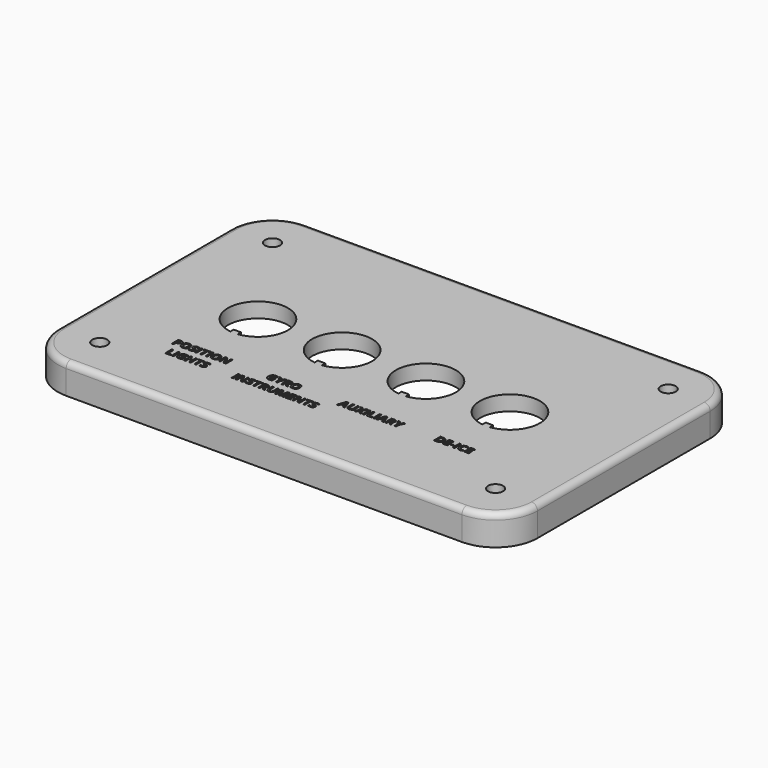
from build123d import *

# Parameters (mm, degrees)
F0_R         = 1.5875
F0_W         = 0.3738893229
F0_H         = 1.7629518229
F0_W_2       = 0.6474574653
F0_H_2       = 0.3013493924
F0_W_3       = 83.82
F0_H_3       = 3.175
F0_TEXT_SIZE = 2.4694444444
F1_DEPTH     = 6.35
F2_R         = 1.27
F3_DEPTH     = 0.508
F5_DEPTH     = 3.175
F6_W         = 83.82
F6_H         = 3.048
F7_DEPTH     = 3.175


# Not quite as in the source:
# - Text() gives the source's letters only with a copy of the font that has no kerning and outlines rounded to 1/6400 em; it was checked with that copy


with BuildPart() as f1:
    # F0 (on Top) → F1 (new body)
    with BuildSketch(Plane.XY):
        with BuildLine():
            Line((-47.7400784737, 22.8871895512), (-47.7400784737, -22.8328104488))
            ThreePointArc((-47.7400784737, -22.8328104488), (-46.0661937282, -26.8739257033), (-42.0250784737, -28.5478104488))
            Line((-42.0250784737, -28.5478104488), (41.7949215263, -28.5478104488))
            ThreePointArc((41.7949215263, -28.5478104488), (45.8360367808, -26.8739257033), (47.5099215263, -22.8328104488))
            Line((47.5099215263, -22.8328104488), (47.5099215263, 22.8871895512))
            ThreePointArc((47.5099215263, 22.8871895512), (45.8360367808, 26.9283048057), (41.7949215263, 28.6021895512))
            Line((41.7949215263, 28.6021895512), (-42.0250784737, 28.6021895512))
            ThreePointArc((-42.0250784737, 28.6021895512), (-46.0661937282, 26.9283048057), (-47.7400784737, 22.8871895512))
        make_face()
        with Locations((-42.0250784737, -22.8328104488)):
            Circle(F0_R, mode=Mode.SUBTRACT)
        Polygon((-30.0736846576, -19.1064444444), (-31.1625553173, -19.1064444444), (-31.1625553173, -17.3434926215), (-30.7886659944, -17.3434926215), (-30.7886659944, -18.7977638889), (-30.0736846576, -18.7977638889), align=None, mode=Mode.SUBTRACT)
        with Locations((-29.5803745447, -18.224968533)):
            Rectangle(F0_W, F0_H, mode=Mode.SUBTRACT)
        with BuildLine():
            Line((-28.2806364805, -18.4277330729), (-28.2806364805, -18.1163515625))
            Line((-28.2806364805, -18.1163515625), (-27.5810891715, -18.1163515625))
            Line((-27.5810891715, -18.1163515625), (-27.5810891715, -19.0304318576))
            add(Edge.make_bspline(
                [(-27.5810891715, -19.0304318576), (-27.7512493277, -19.0859943576), (-27.9013452479, -19.1083736979)],
                knots=[0, 0, 0, 1, 1, 1], degree=2))
            add(Edge.make_bspline(
                [(-27.9013452479, -19.1083736979), (-28.051441168, -19.1307530382), (-28.2080965499, -19.1307530382)],
                knots=[0, 0, 0, 1, 1, 1], degree=2))
            add(Edge.make_bspline(
                [(-28.2080965499, -19.1307530382), (-28.607066168, -19.1307530382), (-28.8175477218, -18.896155816)],
                knots=[0, 0, 0, 1, 1, 1], degree=2))
            add(Edge.make_bspline(
                [(-28.8175477218, -18.896155816), (-29.0280292756, -18.6615585938), (-29.0280292756, -18.2224605035)],
                knots=[0, 0, 0, 1, 1, 1], degree=2))
            add(Edge.make_bspline(
                [(-29.0280292756, -18.2224605035), (-29.0280292756, -17.7957096354), (-28.7837857861, -17.5570609809)],
                knots=[0, 0, 0, 1, 1, 1], degree=2))
            add(Edge.make_bspline(
                [(-28.7837857861, -17.5570609809), (-28.5395422965, -17.3184123264), (-28.107003668, -17.3184123264)],
                knots=[0, 0, 0, 1, 1, 1], degree=2))
            add(Edge.make_bspline(
                [(-28.107003668, -17.3184123264), (-27.8353647791, -17.3184123264), (-27.5834042756, -17.4268363715)],
                knots=[0, 0, 0, 1, 1, 1], degree=2))
            Line((-27.5834042756, -17.4268363715), (-27.7076481993, -17.7258706597))
            add(Edge.make_bspline(
                [(-27.7076481993, -17.7258706597), (-27.9005735465, -17.6294079861), (-28.1093187722, -17.6294079861)],
                knots=[0, 0, 0, 1, 1, 1], degree=2))
            add(Edge.make_bspline(
                [(-28.1093187722, -17.6294079861), (-28.3516330083, -17.6294079861), (-28.4974845708, -17.7922369792)],
                knots=[0, 0, 0, 1, 1, 1], degree=2))
            add(Edge.make_bspline(
                [(-28.4974845708, -17.7922369792), (-28.6433361333, -17.9550659722), (-28.6433361333, -18.2297916667)],
                knots=[0, 0, 0, 1, 1, 1], degree=2))
            add(Edge.make_bspline(
                [(-28.6433361333, -18.2297916667), (-28.6433361333, -18.5168645833), (-28.5258445968, -18.6681180556)],
                knots=[0, 0, 0, 1, 1, 1], degree=2))
            add(Edge.make_bspline(
                [(-28.5258445968, -18.6681180556), (-28.4083530604, -18.8193715278), (-28.1841738069, -18.8193715278)],
                knots=[0, 0, 0, 1, 1, 1], degree=2))
            add(Edge.make_bspline(
                [(-28.1841738069, -18.8193715278), (-28.0668751958, -18.8193715278), (-27.9464897791, -18.7954487847)],
                knots=[0, 0, 0, 1, 1, 1], degree=2))
            Line((-27.9464897791, -18.7954487847), (-27.9464897791, -18.4277330729))
            Line((-27.9464897791, -18.4277330729), (-28.2806364805, -18.4277330729))
        make_face(mode=Mode.SUBTRACT)
        Polygon((-25.7170444666, -17.3434926215), (-25.7170444666, -19.1064444444), (-26.0897762374, -19.1064444444), (-26.0897762374, -18.345546875), (-26.7877801437, -18.345546875), (-26.7877801437, -19.1064444444), (-27.1616694666, -19.1064444444), (-27.1616694666, -17.3434926215), (-26.7877801437, -17.3434926215), (-26.7877801437, -18.0345512153), (-26.0897762374, -18.0345512153), (-26.0897762374, -17.3434926215), align=None, mode=Mode.SUBTRACT)
        Polygon((-24.5919038416, -17.6544882813), (-24.5919038416, -19.1064444444), (-24.9657931645, -19.1064444444), (-24.9657931645, -17.6544882813), (-25.4446338763, -17.6544882813), (-25.4446338763, -17.3434926215), (-24.1134489805, -17.3434926215), (-24.1134489805, -17.6544882813), align=None, mode=Mode.SUBTRACT)
        with BuildLine():
            add(Edge.make_bspline(
                [(-22.8931961593, -18.3256755642), (-22.8015566194, -18.4443246528), (-22.8015566194, -18.6167999132)],
                knots=[0, 0, 0, 1, 1, 1], degree=2))
            add(Edge.make_bspline(
                [(-22.8015566194, -18.6167999132), (-22.8015566194, -18.8556414931), (-22.9734531038, -18.9931972656)],
                knots=[0, 0, 0, 1, 1, 1], degree=2))
            add(Edge.make_bspline(
                [(-22.9734531038, -18.9931972656), (-23.1453495881, -19.1307530382), (-23.4513291888, -19.1307530382)],
                knots=[0, 0, 0, 1, 1, 1], degree=2))
            add(Edge.make_bspline(
                [(-23.4513291888, -19.1307530382), (-23.7337718972, -19.1307530382), (-23.9506199874, -19.0242582465)],
                knots=[0, 0, 0, 1, 1, 1], degree=2))
            Line((-23.9506199874, -19.0242582465), (-23.9506199874, -18.6769926215))
            add(Edge.make_bspline(
                [(-23.9506199874, -18.6769926215), (-23.7723569666, -18.7568637153), (-23.648691819, -18.7892751736)],
                knots=[0, 0, 0, 1, 1, 1], degree=2))
            add(Edge.make_bspline(
                [(-23.648691819, -18.7892751736), (-23.5250266715, -18.8216866319), (-23.4223903868, -18.8216866319)],
                knots=[0, 0, 0, 1, 1, 1], degree=2))
            add(Edge.make_bspline(
                [(-23.4223903868, -18.8216866319), (-23.2996898659, -18.8216866319), (-23.2339023225, -18.7748057726)],
                knots=[0, 0, 0, 1, 1, 1], degree=2))
            add(Edge.make_bspline(
                [(-23.2339023225, -18.7748057726), (-23.1681147791, -18.7279249132), (-23.1681147791, -18.6349348958)],
                knots=[0, 0, 0, 1, 1, 1], degree=2))
            add(Edge.make_bspline(
                [(-23.1681147791, -18.6349348958), (-23.1681147791, -18.5832309028), (-23.1970535812, -18.5427165799)],
                knots=[0, 0, 0, 1, 1, 1], degree=2))
            add(Edge.make_bspline(
                [(-23.1970535812, -18.5427165799), (-23.2259923833, -18.5022022569), (-23.2821336593, -18.4649676649)],
                knots=[0, 0, 0, 1, 1, 1], degree=2))
            add(Edge.make_bspline(
                [(-23.2821336593, -18.4649676649), (-23.3382749354, -18.4277330729), (-23.5107501958, -18.345546875)],
                knots=[0, 0, 0, 1, 1, 1], degree=2))
            add(Edge.make_bspline(
                [(-23.5107501958, -18.345546875), (-23.6720357861, -18.2695342882), (-23.7528715065, -18.1996953125)],
                knots=[0, 0, 0, 1, 1, 1], degree=2))
            add(Edge.make_bspline(
                [(-23.7528715065, -18.1996953125), (-23.833707227, -18.1298563368), (-23.8819385638, -18.0368663194)],
                knots=[0, 0, 0, 1, 1, 1], degree=2))
            add(Edge.make_bspline(
                [(-23.8819385638, -18.0368663194), (-23.9301699006, -17.9438763021), (-23.9301699006, -17.8200182292)],
                knots=[0, 0, 0, 1, 1, 1], degree=2))
            add(Edge.make_bspline(
                [(-23.9301699006, -17.8200182292), (-23.9301699006, -17.5858068576), (-23.7715852652, -17.452109592)],
                knots=[0, 0, 0, 1, 1, 1], degree=2))
            add(Edge.make_bspline(
                [(-23.7715852652, -17.452109592), (-23.6130006298, -17.3184123264), (-23.3332588763, -17.3184123264)],
                knots=[0, 0, 0, 1, 1, 1], degree=2))
            add(Edge.make_bspline(
                [(-23.3332588763, -17.3184123264), (-23.1958960291, -17.3184123264), (-23.0710733295, -17.3508237847)],
                knots=[0, 0, 0, 1, 1, 1], degree=2))
            add(Edge.make_bspline(
                [(-23.0710733295, -17.3508237847), (-22.9462506298, -17.3832352431), (-22.8100453347, -17.4422703993)],
                knots=[0, 0, 0, 1, 1, 1], degree=2))
            Line((-22.8100453347, -17.4422703993), (-22.9304307513, -17.7332018229))
            add(Edge.make_bspline(
                [(-22.9304307513, -17.7332018229), (-23.0716521055, -17.6753242188), (-23.1638704215, -17.6523661024)],
                knots=[0, 0, 0, 1, 1, 1], degree=2))
            add(Edge.make_bspline(
                [(-23.1638704215, -17.6523661024), (-23.2560887374, -17.6294079861), (-23.3452202479, -17.6294079861)],
                knots=[0, 0, 0, 1, 1, 1], degree=2))
            add(Edge.make_bspline(
                [(-23.3452202479, -17.6294079861), (-23.4513291888, -17.6294079861), (-23.5080492409, -17.678796875)],
                knots=[0, 0, 0, 1, 1, 1], degree=2))
            add(Edge.make_bspline(
                [(-23.5080492409, -17.678796875), (-23.564769293, -17.7281857639), (-23.564769293, -17.8076710069)],
                knots=[0, 0, 0, 1, 1, 1], degree=2))
            add(Edge.make_bspline(
                [(-23.564769293, -17.8076710069), (-23.564769293, -17.8570598958), (-23.5418111767, -17.8939086372)],
                knots=[0, 0, 0, 1, 1, 1], degree=2))
            add(Edge.make_bspline(
                [(-23.5418111767, -17.8939086372), (-23.5188530604, -17.9307573785), (-23.4688853954, -17.9650980903)],
                knots=[0, 0, 0, 1, 1, 1], degree=2))
            add(Edge.make_bspline(
                [(-23.4688853954, -17.9650980903), (-23.4189177305, -17.9994388021), (-23.2321659944, -18.0885703125)],
                knots=[0, 0, 0, 1, 1, 1], degree=2))
            add(Edge.make_bspline(
                [(-23.2321659944, -18.0885703125), (-22.9848356993, -18.2070264757), (-22.8931961593, -18.3256755642)],
                knots=[0, 0, 0, 1, 1, 1], degree=2))
        make_face(mode=Mode.SUBTRACT)
        with Locations((-16.8888935736, -18.224968533)):
            Rectangle(F0_W, F0_H, mode=Mode.SUBTRACT)
        with BuildLine():
            Line((-14.694367749, -17.3434926215), (-14.694367749, -19.1064444444))
            Line((-14.694367749, -19.1064444444), (-15.1693499538, -19.1064444444))
            Line((-15.1693499538, -19.1064444444), (-15.9364211344, -17.7729444444))
            Line((-15.9364211344, -17.7729444444), (-15.9472249538, -17.7729444444))
            add(Edge.make_bspline(
                [(-15.9472249538, -17.7729444444), (-15.9240739122, -18.1259978299), (-15.9240739122, -18.2768654514)],
                knots=[0, 0, 0, 1, 1, 1], degree=2))
            Line((-15.9240739122, -18.2768654514), (-15.9240739122, -19.1064444444))
            Line((-15.9240739122, -19.1064444444), (-16.2582206136, -19.1064444444))
            Line((-16.2582206136, -19.1064444444), (-16.2582206136, -17.3434926215))
            Line((-16.2582206136, -17.3434926215), (-15.7867110649, -17.3434926215))
            Line((-15.7867110649, -17.3434926215), (-15.0211832872, -18.6638736979))
            Line((-15.0211832872, -18.6638736979), (-15.0126945719, -18.6638736979))
            add(Edge.make_bspline(
                [(-15.0126945719, -18.6638736979), (-15.0308295545, -18.3200807292), (-15.0308295545, -18.1780876736)],
                knots=[0, 0, 0, 1, 1, 1], degree=2))
            Line((-15.0308295545, -18.1780876736), (-15.0308295545, -17.3434926215))
            Line((-15.0308295545, -17.3434926215), (-14.694367749, -17.3434926215))
        make_face(mode=Mode.SUBTRACT)
        with BuildLine():
            add(Edge.make_bspline(
                [(-13.3016396674, -18.3256755642), (-13.2100001274, -18.4443246528), (-13.2100001274, -18.6167999132)],
                knots=[0, 0, 0, 1, 1, 1], degree=2))
            add(Edge.make_bspline(
                [(-13.2100001274, -18.6167999132), (-13.2100001274, -18.8556414931), (-13.3818966118, -18.9931972656)],
                knots=[0, 0, 0, 1, 1, 1], degree=2))
            add(Edge.make_bspline(
                [(-13.3818966118, -18.9931972656), (-13.5537930962, -19.1307530382), (-13.8597726969, -19.1307530382)],
                knots=[0, 0, 0, 1, 1, 1], degree=2))
            add(Edge.make_bspline(
                [(-13.8597726969, -19.1307530382), (-14.1422154052, -19.1307530382), (-14.3590634955, -19.0242582465)],
                knots=[0, 0, 0, 1, 1, 1], degree=2))
            Line((-14.3590634955, -19.0242582465), (-14.3590634955, -18.6769926215))
            add(Edge.make_bspline(
                [(-14.3590634955, -18.6769926215), (-14.1808004747, -18.7568637153), (-14.0571353271, -18.7892751736)],
                knots=[0, 0, 0, 1, 1, 1], degree=2))
            add(Edge.make_bspline(
                [(-14.0571353271, -18.7892751736), (-13.9334701795, -18.8216866319), (-13.8308338948, -18.8216866319)],
                knots=[0, 0, 0, 1, 1, 1], degree=2))
            add(Edge.make_bspline(
                [(-13.8308338948, -18.8216866319), (-13.708133374, -18.8216866319), (-13.6423458306, -18.7748057726)],
                knots=[0, 0, 0, 1, 1, 1], degree=2))
            add(Edge.make_bspline(
                [(-13.6423458306, -18.7748057726), (-13.5765582872, -18.7279249132), (-13.5765582872, -18.6349348958)],
                knots=[0, 0, 0, 1, 1, 1], degree=2))
            add(Edge.make_bspline(
                [(-13.5765582872, -18.6349348958), (-13.5765582872, -18.5832309028), (-13.6054970893, -18.5427165799)],
                knots=[0, 0, 0, 1, 1, 1], degree=2))
            add(Edge.make_bspline(
                [(-13.6054970893, -18.5427165799), (-13.6344358913, -18.5022022569), (-13.6905771674, -18.4649676649)],
                knots=[0, 0, 0, 1, 1, 1], degree=2))
            add(Edge.make_bspline(
                [(-13.6905771674, -18.4649676649), (-13.7467184434, -18.4277330729), (-13.9191937038, -18.345546875)],
                knots=[0, 0, 0, 1, 1, 1], degree=2))
            add(Edge.make_bspline(
                [(-13.9191937038, -18.345546875), (-14.0804792941, -18.2695342882), (-14.1613150146, -18.1996953125)],
                knots=[0, 0, 0, 1, 1, 1], degree=2))
            add(Edge.make_bspline(
                [(-14.1613150146, -18.1996953125), (-14.2421507351, -18.1298563368), (-14.2903820719, -18.0368663194)],
                knots=[0, 0, 0, 1, 1, 1], degree=2))
            add(Edge.make_bspline(
                [(-14.2903820719, -18.0368663194), (-14.3386134087, -17.9438763021), (-14.3386134087, -17.8200182292)],
                knots=[0, 0, 0, 1, 1, 1], degree=2))
            add(Edge.make_bspline(
                [(-14.3386134087, -17.8200182292), (-14.3386134087, -17.5858068576), (-14.1800287733, -17.452109592)],
                knots=[0, 0, 0, 1, 1, 1], degree=2))
            add(Edge.make_bspline(
                [(-14.1800287733, -17.452109592), (-14.0214441379, -17.3184123264), (-13.7417023844, -17.3184123264)],
                knots=[0, 0, 0, 1, 1, 1], degree=2))
            add(Edge.make_bspline(
                [(-13.7417023844, -17.3184123264), (-13.6043395372, -17.3184123264), (-13.4795168375, -17.3508237847)],
                knots=[0, 0, 0, 1, 1, 1], degree=2))
            add(Edge.make_bspline(
                [(-13.4795168375, -17.3508237847), (-13.3546941379, -17.3832352431), (-13.2184888427, -17.4422703993)],
                knots=[0, 0, 0, 1, 1, 1], degree=2))
            Line((-13.2184888427, -17.4422703993), (-13.3388742594, -17.7332018229))
            add(Edge.make_bspline(
                [(-13.3388742594, -17.7332018229), (-13.4800956136, -17.6753242188), (-13.5723139295, -17.6523661024)],
                knots=[0, 0, 0, 1, 1, 1], degree=2))
            add(Edge.make_bspline(
                [(-13.5723139295, -17.6523661024), (-13.6645322455, -17.6294079861), (-13.7536637559, -17.6294079861)],
                knots=[0, 0, 0, 1, 1, 1], degree=2))
            add(Edge.make_bspline(
                [(-13.7536637559, -17.6294079861), (-13.8597726969, -17.6294079861), (-13.916492749, -17.678796875)],
                knots=[0, 0, 0, 1, 1, 1], degree=2))
            add(Edge.make_bspline(
                [(-13.916492749, -17.678796875), (-13.9732128011, -17.7281857639), (-13.9732128011, -17.8076710069)],
                knots=[0, 0, 0, 1, 1, 1], degree=2))
            add(Edge.make_bspline(
                [(-13.9732128011, -17.8076710069), (-13.9732128011, -17.8570598958), (-13.9502546847, -17.8939086372)],
                knots=[0, 0, 0, 1, 1, 1], degree=2))
            add(Edge.make_bspline(
                [(-13.9502546847, -17.8939086372), (-13.9272965684, -17.9307573785), (-13.8773289035, -17.9650980903)],
                knots=[0, 0, 0, 1, 1, 1], degree=2))
            add(Edge.make_bspline(
                [(-13.8773289035, -17.9650980903), (-13.8273612386, -17.9994388021), (-13.6406095024, -18.0885703125)],
                knots=[0, 0, 0, 1, 1, 1], degree=2))
            add(Edge.make_bspline(
                [(-13.6406095024, -18.0885703125), (-13.3932792073, -18.2070264757), (-13.3016396674, -18.3256755642)],
                knots=[0, 0, 0, 1, 1, 1], degree=2))
        make_face(mode=Mode.SUBTRACT)
        Polygon((-12.2102609781, -17.6544882813), (-12.2102609781, -19.1064444444), (-12.5841503011, -19.1064444444), (-12.5841503011, -17.6544882813), (-13.0629910129, -17.6544882813), (-13.0629910129, -17.3434926215), (-11.731806117, -17.3434926215), (-11.731806117, -17.6544882813), align=None, mode=Mode.SUBTRACT)
        with BuildLine():
            Line((-10.8879506483, -18.4300481771), (-11.0866637559, -18.4300481771))
            Line((-11.0866637559, -18.4300481771), (-11.0866637559, -19.1064444444))
            Line((-11.0866637559, -19.1064444444), (-11.4605530788, -19.1064444444))
            Line((-11.4605530788, -19.1064444444), (-11.4605530788, -17.3434926215))
            Line((-11.4605530788, -17.3434926215), (-10.9469858045, -17.3434926215))
            add(Edge.make_bspline(
                [(-10.9469858045, -17.3434926215), (-10.5873729573, -17.3434926215), (-10.4150906222, -17.4742960069)],
                knots=[0, 0, 0, 1, 1, 1], degree=2))
            add(Edge.make_bspline(
                [(-10.4150906222, -17.4742960069), (-10.2428082872, -17.6050993924), (-10.2428082872, -17.8717222222)],
                knots=[0, 0, 0, 1, 1, 1], degree=2))
            add(Edge.make_bspline(
                [(-10.2428082872, -17.8717222222), (-10.2428082872, -18.0272200521), (-10.328274216, -18.1483771701)],
                knots=[0, 0, 0, 1, 1, 1], degree=2))
            add(Edge.make_bspline(
                [(-10.328274216, -18.1483771701), (-10.4137401448, -18.2695342882), (-10.5707813774, -18.3382157118)],
                knots=[0, 0, 0, 1, 1, 1], degree=2))
            add(Edge.make_bspline(
                [(-10.5707813774, -18.3382157118), (-10.1725834608, -18.9328116319), (-10.0521980441, -19.1064444444)],
                knots=[0, 0, 0, 1, 1, 1], degree=2))
            Line((-10.0521980441, -19.1064444444), (-10.4669875406, -19.1064444444))
            Line((-10.4669875406, -19.1064444444), (-10.8879506483, -18.4300481771))
        make_face(mode=Mode.SUBTRACT)
        with BuildLine():
            Line((-8.768086933, -17.3434926215), (-8.3953551622, -17.3434926215))
            Line((-8.3953551622, -17.3434926215), (-8.3953551622, -18.4840672743))
            add(Edge.make_bspline(
                [(-8.3953551622, -18.4840672743), (-8.3953551622, -18.6796935764), (-8.4827503445, -18.826702691)],
                knots=[0, 0, 0, 1, 1, 1], degree=2))
            add(Edge.make_bspline(
                [(-8.4827503445, -18.826702691), (-8.5701455268, -18.9737118056), (-8.7354825493, -19.0522324219)],
                knots=[0, 0, 0, 1, 1, 1], degree=2))
            add(Edge.make_bspline(
                [(-8.7354825493, -19.0522324219), (-8.9008195719, -19.1307530382), (-9.1261563774, -19.1307530382)],
                knots=[0, 0, 0, 1, 1, 1], degree=2))
            add(Edge.make_bspline(
                [(-9.1261563774, -19.1307530382), (-9.4660908393, -19.1307530382), (-9.6541930528, -18.9563485243)],
                knots=[0, 0, 0, 1, 1, 1], degree=2))
            add(Edge.make_bspline(
                [(-9.6541930528, -18.9563485243), (-9.8422952663, -18.7819440104), (-9.8422952663, -18.479437066)],
                knots=[0, 0, 0, 1, 1, 1], degree=2))
            Line((-9.8422952663, -18.479437066), (-9.8422952663, -17.3434926215))
            Line((-9.8422952663, -17.3434926215), (-9.4699493462, -17.3434926215))
            Line((-9.4699493462, -17.3434926215), (-9.4699493462, -18.4227170139))
            add(Edge.make_bspline(
                [(-9.4699493462, -18.4227170139), (-9.4699493462, -18.6264461806), (-9.3879560736, -18.7217513021)],
                knots=[0, 0, 0, 1, 1, 1], degree=2))
            add(Edge.make_bspline(
                [(-9.3879560736, -18.7217513021), (-9.3059628011, -18.8170564236), (-9.1165101101, -18.8170564236)],
                knots=[0, 0, 0, 1, 1, 1], degree=2))
            add(Edge.make_bspline(
                [(-9.1165101101, -18.8170564236), (-8.9332310302, -18.8170564236), (-8.8506589816, -18.721172526)],
                knots=[0, 0, 0, 1, 1, 1], degree=2))
            add(Edge.make_bspline(
                [(-8.8506589816, -18.721172526), (-8.768086933, -18.6252886285), (-8.768086933, -18.4204019097)],
                knots=[0, 0, 0, 1, 1, 1], degree=2))
            Line((-8.768086933, -18.4204019097), (-8.768086933, -17.3434926215))
        make_face(mode=Mode.SUBTRACT)
        with BuildLine():
            Line((-6.8747175754, -19.1064444444), (-7.217352992, -19.1064444444))
            Line((-7.217352992, -19.1064444444), (-7.6417887559, -17.7235555556))
            Line((-7.6417887559, -17.7235555556), (-7.6525925754, -17.7235555556))
            add(Edge.make_bspline(
                [(-7.6525925754, -17.7235555556), (-7.6294415337, -18.1452903646), (-7.6294415337, -18.2865117188)],
                knots=[0, 0, 0, 1, 1, 1], degree=2))
            Line((-7.6294415337, -18.2865117188), (-7.6294415337, -19.1064444444))
            Line((-7.6294415337, -19.1064444444), (-7.9635882351, -19.1064444444))
            Line((-7.9635882351, -19.1064444444), (-7.9635882351, -17.3434926215))
            Line((-7.9635882351, -17.3434926215), (-7.4546511691, -17.3434926215))
            Line((-7.4546511691, -17.3434926215), (-7.0375465684, -18.6916549479))
            Line((-7.0375465684, -18.6916549479), (-7.0302154052, -18.6916549479))
            Line((-7.0302154052, -18.6916549479), (-6.5876446587, -17.3434926215))
            Line((-6.5876446587, -17.3434926215), (-6.0790934434, -17.3434926215))
            Line((-6.0790934434, -17.3434926215), (-6.0790934434, -19.1064444444))
            Line((-6.0790934434, -19.1064444444), (-6.4275166205, -19.1064444444))
            Line((-6.4275166205, -19.1064444444), (-6.4275166205, -18.2718493924))
            add(Edge.make_bspline(
                [(-6.4275166205, -18.2718493924), (-6.4275166205, -18.2128142361), (-6.425587367, -18.1356440972)],
                knots=[0, 0, 0, 1, 1, 1], degree=2))
            add(Edge.make_bspline(
                [(-6.425587367, -18.1356440972), (-6.4236581136, -18.0584739583), (-6.4093816379, -17.7258706597)],
                knots=[0, 0, 0, 1, 1, 1], degree=2))
            Line((-6.4093816379, -17.7258706597), (-6.4201854573, -17.7258706597))
            Line((-6.4201854573, -17.7258706597), (-6.8747175754, -19.1064444444))
        make_face(mode=Mode.SUBTRACT)
        Polygon((-4.6201919677, -18.7977638889), (-4.6201919677, -19.1064444444), (-5.6353651448, -19.1064444444), (-5.6353651448, -17.3434926215), (-4.6201919677, -17.3434926215), (-4.6201919677, -17.6498580729), (-5.2614758219, -17.6498580729), (-5.2614758219, -18.0368663194), (-4.6645647976, -18.0368663194), (-4.6645647976, -18.3432317708), (-5.2614758219, -18.3432317708), (-5.2614758219, -18.7977638889), align=None, mode=Mode.SUBTRACT)
        with BuildLine():
            Line((-2.6886233913, -17.3434926215), (-2.6886233913, -19.1064444444))
            Line((-2.6886233913, -19.1064444444), (-3.1636055962, -19.1064444444))
            Line((-3.1636055962, -19.1064444444), (-3.9306767768, -17.7729444444))
            Line((-3.9306767768, -17.7729444444), (-3.9414805962, -17.7729444444))
            add(Edge.make_bspline(
                [(-3.9414805962, -17.7729444444), (-3.9183295545, -18.1259978299), (-3.9183295545, -18.2768654514)],
                knots=[0, 0, 0, 1, 1, 1], degree=2))
            Line((-3.9183295545, -18.2768654514), (-3.9183295545, -19.1064444444))
            Line((-3.9183295545, -19.1064444444), (-4.2524762559, -19.1064444444))
            Line((-4.2524762559, -19.1064444444), (-4.2524762559, -17.3434926215))
            Line((-4.2524762559, -17.3434926215), (-3.7809667073, -17.3434926215))
            Line((-3.7809667073, -17.3434926215), (-3.0154389295, -18.6638736979))
            Line((-3.0154389295, -18.6638736979), (-3.0069502143, -18.6638736979))
            add(Edge.make_bspline(
                [(-3.0069502143, -18.6638736979), (-3.0250851969, -18.3200807292), (-3.0250851969, -18.1780876736)],
                knots=[0, 0, 0, 1, 1, 1], degree=2))
            Line((-3.0250851969, -18.1780876736), (-3.0250851969, -17.3434926215))
            Line((-3.0250851969, -17.3434926215), (-2.6886233913, -17.3434926215))
        make_face(mode=Mode.SUBTRACT)
        Polygon((-1.5646403184, -17.6544882813), (-1.5646403184, -19.1064444444), (-1.9385296413, -19.1064444444), (-1.9385296413, -17.6544882813), (-2.4173703531, -17.6544882813), (-2.4173703531, -17.3434926215), (-1.0861854573, -17.3434926215), (-1.0861854573, -17.6544882813), align=None, mode=Mode.SUBTRACT)
        with BuildLine():
            add(Edge.make_bspline(
                [(0.1340673639, -18.3256755642), (0.2257069038, -18.4443246528), (0.2257069038, -18.6167999132)],
                knots=[0, 0, 0, 1, 1, 1], degree=2))
            add(Edge.make_bspline(
                [(0.2257069038, -18.6167999132), (0.2257069038, -18.8556414931), (0.0538104194, -18.9931972656)],
                knots=[0, 0, 0, 1, 1, 1], degree=2))
            add(Edge.make_bspline(
                [(0.0538104194, -18.9931972656), (-0.1180860649, -19.1307530382), (-0.4240656656, -19.1307530382)],
                knots=[0, 0, 0, 1, 1, 1], degree=2))
            add(Edge.make_bspline(
                [(-0.4240656656, -19.1307530382), (-0.706508374, -19.1307530382), (-0.9233564643, -19.0242582465)],
                knots=[0, 0, 0, 1, 1, 1], degree=2))
            Line((-0.9233564643, -19.0242582465), (-0.9233564643, -18.6769926215))
            add(Edge.make_bspline(
                [(-0.9233564643, -18.6769926215), (-0.7450934434, -18.7568637153), (-0.6214282959, -18.7892751736)],
                knots=[0, 0, 0, 1, 1, 1], degree=2))
            add(Edge.make_bspline(
                [(-0.6214282959, -18.7892751736), (-0.4977631483, -18.8216866319), (-0.3951268636, -18.8216866319)],
                knots=[0, 0, 0, 1, 1, 1], degree=2))
            add(Edge.make_bspline(
                [(-0.3951268636, -18.8216866319), (-0.2724263427, -18.8216866319), (-0.2066387993, -18.7748057726)],
                knots=[0, 0, 0, 1, 1, 1], degree=2))
            add(Edge.make_bspline(
                [(-0.2066387993, -18.7748057726), (-0.1408512559, -18.7279249132), (-0.1408512559, -18.6349348958)],
                knots=[0, 0, 0, 1, 1, 1], degree=2))
            add(Edge.make_bspline(
                [(-0.1408512559, -18.6349348958), (-0.1408512559, -18.5832309028), (-0.169790058, -18.5427165799)],
                knots=[0, 0, 0, 1, 1, 1], degree=2))
            add(Edge.make_bspline(
                [(-0.169790058, -18.5427165799), (-0.1987288601, -18.5022022569), (-0.2548701361, -18.4649676649)],
                knots=[0, 0, 0, 1, 1, 1], degree=2))
            add(Edge.make_bspline(
                [(-0.2548701361, -18.4649676649), (-0.3110114122, -18.4277330729), (-0.4834866726, -18.345546875)],
                knots=[0, 0, 0, 1, 1, 1], degree=2))
            add(Edge.make_bspline(
                [(-0.4834866726, -18.345546875), (-0.6447722629, -18.2695342882), (-0.7256079834, -18.1996953125)],
                knots=[0, 0, 0, 1, 1, 1], degree=2))
            add(Edge.make_bspline(
                [(-0.7256079834, -18.1996953125), (-0.8064437038, -18.1298563368), (-0.8546750406, -18.0368663194)],
                knots=[0, 0, 0, 1, 1, 1], degree=2))
            add(Edge.make_bspline(
                [(-0.8546750406, -18.0368663194), (-0.9029063774, -17.9438763021), (-0.9029063774, -17.8200182292)],
                knots=[0, 0, 0, 1, 1, 1], degree=2))
            add(Edge.make_bspline(
                [(-0.9029063774, -17.8200182292), (-0.9029063774, -17.5858068576), (-0.744321742, -17.452109592)],
                knots=[0, 0, 0, 1, 1, 1], degree=2))
            add(Edge.make_bspline(
                [(-0.744321742, -17.452109592), (-0.5857371066, -17.3184123264), (-0.3059953531, -17.3184123264)],
                knots=[0, 0, 0, 1, 1, 1], degree=2))
            add(Edge.make_bspline(
                [(-0.3059953531, -17.3184123264), (-0.1686325059, -17.3184123264), (-0.0438098063, -17.3508237847)],
                knots=[0, 0, 0, 1, 1, 1], degree=2))
            add(Edge.make_bspline(
                [(-0.0438098063, -17.3508237847), (0.0810128934, -17.3832352431), (0.2172181885, -17.4422703993)],
                knots=[0, 0, 0, 1, 1, 1], degree=2))
            Line((0.2172181885, -17.4422703993), (0.0968327719, -17.7332018229))
            add(Edge.make_bspline(
                [(0.0968327719, -17.7332018229), (-0.0443885823, -17.6753242188), (-0.1366068983, -17.6523661024)],
                knots=[0, 0, 0, 1, 1, 1], degree=2))
            add(Edge.make_bspline(
                [(-0.1366068983, -17.6523661024), (-0.2288252143, -17.6294079861), (-0.3179567247, -17.6294079861)],
                knots=[0, 0, 0, 1, 1, 1], degree=2))
            add(Edge.make_bspline(
                [(-0.3179567247, -17.6294079861), (-0.4240656656, -17.6294079861), (-0.4807857177, -17.678796875)],
                knots=[0, 0, 0, 1, 1, 1], degree=2))
            add(Edge.make_bspline(
                [(-0.4807857177, -17.678796875), (-0.5375057698, -17.7281857639), (-0.5375057698, -17.8076710069)],
                knots=[0, 0, 0, 1, 1, 1], degree=2))
            add(Edge.make_bspline(
                [(-0.5375057698, -17.8076710069), (-0.5375057698, -17.8570598958), (-0.5145476535, -17.8939086372)],
                knots=[0, 0, 0, 1, 1, 1], degree=2))
            add(Edge.make_bspline(
                [(-0.5145476535, -17.8939086372), (-0.4915895372, -17.9307573785), (-0.4416218722, -17.9650980903)],
                knots=[0, 0, 0, 1, 1, 1], degree=2))
            add(Edge.make_bspline(
                [(-0.4416218722, -17.9650980903), (-0.3916542073, -17.9994388021), (-0.2049024712, -18.0885703125)],
                knots=[0, 0, 0, 1, 1, 1], degree=2))
            add(Edge.make_bspline(
                [(-0.2049024712, -18.0885703125), (0.0424278239, -18.2070264757), (0.1340673639, -18.3256755642)],
                knots=[0, 0, 0, 1, 1, 1], degree=2))
        make_face(mode=Mode.SUBTRACT)
        with BuildLine():
            add(Edge.make_bspline(
                [(-31.3950303607, -14.1231827257), (-31.2281499354, -14.2613172743), (-31.2281499354, -14.5348854167)],
                knots=[0, 0, 0, 1, 1, 1], degree=2))
            add(Edge.make_bspline(
                [(-31.2281499354, -14.5348854167), (-31.2281499354, -14.8196432292), (-31.4060271055, -14.9703179253)],
                knots=[0, 0, 0, 1, 1, 1], degree=2))
            add(Edge.make_bspline(
                [(-31.4060271055, -14.9703179253), (-31.5839042756, -15.1209926215), (-31.9118773659, -15.1209926215)],
                knots=[0, 0, 0, 1, 1, 1], degree=2))
            Line((-31.9118773659, -15.1209926215), (-32.0720054041, -15.1209926215))
            Line((-32.0720054041, -15.1209926215), (-32.0720054041, -15.748))
            Line((-32.0720054041, -15.748), (-32.445894727, -15.748))
            Line((-32.445894727, -15.748), (-32.445894727, -13.9850481771))
            Line((-32.445894727, -13.9850481771), (-31.8829385638, -13.9850481771))
            add(Edge.make_bspline(
                [(-31.8829385638, -13.9850481771), (-31.5619107861, -13.9850481771), (-31.3950303607, -14.1231827257)],
                knots=[0, 0, 0, 1, 1, 1], degree=2))
        make_face(mode=Mode.SUBTRACT)
        with BuildLine():
            add(Edge.make_bspline(
                [(-29.5103426437, -14.1912853733), (-29.2950379562, -14.4253038194), (-29.2950379562, -14.864016059)],
                knots=[0, 0, 0, 1, 1, 1], degree=2))
            add(Edge.make_bspline(
                [(-29.2950379562, -14.864016059), (-29.2950379562, -15.3019565972), (-29.5120789718, -15.5371325955)],
                knots=[0, 0, 0, 1, 1, 1], degree=2))
            add(Edge.make_bspline(
                [(-29.5120789718, -15.5371325955), (-29.7291199874, -15.7723085938), (-30.1342632166, -15.7723085938)],
                knots=[0, 0, 0, 1, 1, 1], degree=2))
            add(Edge.make_bspline(
                [(-30.1342632166, -15.7723085938), (-30.5394064458, -15.7723085938), (-30.7564474614, -15.5371325955)],
                knots=[0, 0, 0, 1, 1, 1], degree=2))
            add(Edge.make_bspline(
                [(-30.7564474614, -15.5371325955), (-30.973488477, -15.3019565972), (-30.973488477, -14.8617009549)],
                knots=[0, 0, 0, 1, 1, 1], degree=2))
            add(Edge.make_bspline(
                [(-30.973488477, -14.8617009549), (-30.973488477, -14.4214453125), (-30.7558686854, -14.1893561198)],
                knots=[0, 0, 0, 1, 1, 1], degree=2))
            add(Edge.make_bspline(
                [(-30.7558686854, -14.1893561198), (-30.5382488937, -13.9572669271), (-30.1319481124, -13.9572669271)],
                knots=[0, 0, 0, 1, 1, 1], degree=2))
            add(Edge.make_bspline(
                [(-30.1319481124, -13.9572669271), (-29.7256473312, -13.9572669271), (-29.5103426437, -14.1912853733)],
                knots=[0, 0, 0, 1, 1, 1], degree=2))
        make_face(mode=Mode.SUBTRACT)
        with BuildLine():
            add(Edge.make_bspline(
                [(-27.9806375656, -14.9672311198), (-27.8889980256, -15.0858802083), (-27.8889980256, -15.2583554688)],
                knots=[0, 0, 0, 1, 1, 1], degree=2))
            add(Edge.make_bspline(
                [(-27.8889980256, -15.2583554688), (-27.8889980256, -15.4971970486), (-28.06089451, -15.6347528212)],
                knots=[0, 0, 0, 1, 1, 1], degree=2))
            add(Edge.make_bspline(
                [(-28.06089451, -15.6347528212), (-28.2327909944, -15.7723085938), (-28.5387705951, -15.7723085938)],
                knots=[0, 0, 0, 1, 1, 1], degree=2))
            add(Edge.make_bspline(
                [(-28.5387705951, -15.7723085938), (-28.8212133034, -15.7723085938), (-29.0380613937, -15.6658138021)],
                knots=[0, 0, 0, 1, 1, 1], degree=2))
            Line((-29.0380613937, -15.6658138021), (-29.0380613937, -15.3185481771))
            add(Edge.make_bspline(
                [(-29.0380613937, -15.3185481771), (-28.8597983729, -15.3984192708), (-28.7361332253, -15.4308307292)],
                knots=[0, 0, 0, 1, 1, 1], degree=2))
            add(Edge.make_bspline(
                [(-28.7361332253, -15.4308307292), (-28.6124680777, -15.4632421875), (-28.509831793, -15.4632421875)],
                knots=[0, 0, 0, 1, 1, 1], degree=2))
            add(Edge.make_bspline(
                [(-28.509831793, -15.4632421875), (-28.3871312722, -15.4632421875), (-28.3213437288, -15.4163613281)],
                knots=[0, 0, 0, 1, 1, 1], degree=2))
            add(Edge.make_bspline(
                [(-28.3213437288, -15.4163613281), (-28.2555561854, -15.3694804688), (-28.2555561854, -15.2764904514)],
                knots=[0, 0, 0, 1, 1, 1], degree=2))
            add(Edge.make_bspline(
                [(-28.2555561854, -15.2764904514), (-28.2555561854, -15.2247864583), (-28.2844949874, -15.1842721354)],
                knots=[0, 0, 0, 1, 1, 1], degree=2))
            add(Edge.make_bspline(
                [(-28.2844949874, -15.1842721354), (-28.3134337895, -15.1437578125), (-28.3695750656, -15.1065232205)],
                knots=[0, 0, 0, 1, 1, 1], degree=2))
            add(Edge.make_bspline(
                [(-28.3695750656, -15.1065232205), (-28.4257163416, -15.0692886285), (-28.598191602, -14.9871024306)],
                knots=[0, 0, 0, 1, 1, 1], degree=2))
            add(Edge.make_bspline(
                [(-28.598191602, -14.9871024306), (-28.7594771923, -14.9110898438), (-28.8403129128, -14.8412508681)],
                knots=[0, 0, 0, 1, 1, 1], degree=2))
            add(Edge.make_bspline(
                [(-28.8403129128, -14.8412508681), (-28.9211486333, -14.7714118924), (-28.9693799701, -14.678421875)],
                knots=[0, 0, 0, 1, 1, 1], degree=2))
            add(Edge.make_bspline(
                [(-28.9693799701, -14.678421875), (-29.0176113069, -14.5854318576), (-29.0176113069, -14.4615737847)],
                knots=[0, 0, 0, 1, 1, 1], degree=2))
            add(Edge.make_bspline(
                [(-29.0176113069, -14.4615737847), (-29.0176113069, -14.2273624132), (-28.8590266715, -14.0936651476)],
                knots=[0, 0, 0, 1, 1, 1], degree=2))
            add(Edge.make_bspline(
                [(-28.8590266715, -14.0936651476), (-28.7004420361, -13.9599678819), (-28.4207002826, -13.9599678819)],
                knots=[0, 0, 0, 1, 1, 1], degree=2))
            add(Edge.make_bspline(
                [(-28.4207002826, -13.9599678819), (-28.2833374354, -13.9599678819), (-28.1585147357, -13.9923793403)],
                knots=[0, 0, 0, 1, 1, 1], degree=2))
            add(Edge.make_bspline(
                [(-28.1585147357, -13.9923793403), (-28.0336920361, -14.0247907986), (-27.8974867409, -14.0838259549)],
                knots=[0, 0, 0, 1, 1, 1], degree=2))
            Line((-27.8974867409, -14.0838259549), (-28.0178721576, -14.3747573785))
            add(Edge.make_bspline(
                [(-28.0178721576, -14.3747573785), (-28.1590935118, -14.3168797743), (-28.2513118277, -14.293921658)],
                knots=[0, 0, 0, 1, 1, 1], degree=2))
            add(Edge.make_bspline(
                [(-28.2513118277, -14.293921658), (-28.3435301437, -14.2709635417), (-28.4326616541, -14.2709635417)],
                knots=[0, 0, 0, 1, 1, 1], degree=2))
            add(Edge.make_bspline(
                [(-28.4326616541, -14.2709635417), (-28.5387705951, -14.2709635417), (-28.5954906472, -14.3203524306)],
                knots=[0, 0, 0, 1, 1, 1], degree=2))
            add(Edge.make_bspline(
                [(-28.5954906472, -14.3203524306), (-28.6522106993, -14.3697413194), (-28.6522106993, -14.4492265625)],
                knots=[0, 0, 0, 1, 1, 1], degree=2))
            add(Edge.make_bspline(
                [(-28.6522106993, -14.4492265625), (-28.6522106993, -14.4986154514), (-28.6292525829, -14.5354641927)],
                knots=[0, 0, 0, 1, 1, 1], degree=2))
            add(Edge.make_bspline(
                [(-28.6292525829, -14.5354641927), (-28.6062944666, -14.572312934), (-28.5563268017, -14.6066536458)],
                knots=[0, 0, 0, 1, 1, 1], degree=2))
            add(Edge.make_bspline(
                [(-28.5563268017, -14.6066536458), (-28.5063591368, -14.6409943576), (-28.3196074006, -14.7301258681)],
                knots=[0, 0, 0, 1, 1, 1], degree=2))
            add(Edge.make_bspline(
                [(-28.3196074006, -14.7301258681), (-28.0722771055, -14.8485820313), (-27.9806375656, -14.9672311198)],
                knots=[0, 0, 0, 1, 1, 1], degree=2))
        make_face(mode=Mode.SUBTRACT)
        with Locations((-27.3825689892, -14.8665240885)):
            Rectangle(F0_W, F0_H, mode=Mode.SUBTRACT)
        Polygon((-26.0716412548, -14.2960438368), (-26.0716412548, -15.748), (-26.4455305777, -15.748), (-26.4455305777, -14.2960438368), (-26.9243712895, -14.2960438368), (-26.9243712895, -13.9850481771), (-25.5931863937, -13.9850481771), (-25.5931863937, -14.2960438368), align=None, mode=Mode.SUBTRACT)
        with Locations((-25.134988694, -14.8665240885)):
            Rectangle(F0_W, F0_H, mode=Mode.SUBTRACT)
        with BuildLine():
            add(Edge.make_bspline(
                [(-23.1194975916, -14.1912853733), (-22.9041929041, -14.4253038194), (-22.9041929041, -14.864016059)],
                knots=[0, 0, 0, 1, 1, 1], degree=2))
            add(Edge.make_bspline(
                [(-22.9041929041, -14.864016059), (-22.9041929041, -15.3019565972), (-23.1212339197, -15.5371325955)],
                knots=[0, 0, 0, 1, 1, 1], degree=2))
            add(Edge.make_bspline(
                [(-23.1212339197, -15.5371325955), (-23.3382749354, -15.7723085938), (-23.7434181645, -15.7723085938)],
                knots=[0, 0, 0, 1, 1, 1], degree=2))
            add(Edge.make_bspline(
                [(-23.7434181645, -15.7723085938), (-24.1485613937, -15.7723085938), (-24.3656024093, -15.5371325955)],
                knots=[0, 0, 0, 1, 1, 1], degree=2))
            add(Edge.make_bspline(
                [(-24.3656024093, -15.5371325955), (-24.5826434249, -15.3019565972), (-24.5826434249, -14.8617009549)],
                knots=[0, 0, 0, 1, 1, 1], degree=2))
            add(Edge.make_bspline(
                [(-24.5826434249, -14.8617009549), (-24.5826434249, -14.4214453125), (-24.3650236333, -14.1893561198)],
                knots=[0, 0, 0, 1, 1, 1], degree=2))
            add(Edge.make_bspline(
                [(-24.3650236333, -14.1893561198), (-24.1474038416, -13.9572669271), (-23.7411030604, -13.9572669271)],
                knots=[0, 0, 0, 1, 1, 1], degree=2))
            add(Edge.make_bspline(
                [(-23.7411030604, -13.9572669271), (-23.3348022791, -13.9572669271), (-23.1194975916, -14.1912853733)],
                knots=[0, 0, 0, 1, 1, 1], degree=2))
        make_face(mode=Mode.SUBTRACT)
        with BuildLine():
            Line((-20.9749394319, -13.9850481771), (-20.9749394319, -15.748))
            Line((-20.9749394319, -15.748), (-21.4499216368, -15.748))
            Line((-21.4499216368, -15.748), (-22.2169928173, -14.4145))
            Line((-22.2169928173, -14.4145), (-22.2277966368, -14.4145))
            add(Edge.make_bspline(
                [(-22.2277966368, -14.4145), (-22.2046455951, -14.7675533854), (-22.2046455951, -14.9184210069)],
                knots=[0, 0, 0, 1, 1, 1], degree=2))
            Line((-22.2046455951, -14.9184210069), (-22.2046455951, -15.748))
            Line((-22.2046455951, -15.748), (-22.5387922965, -15.748))
            Line((-22.5387922965, -15.748), (-22.5387922965, -13.9850481771))
            Line((-22.5387922965, -13.9850481771), (-22.0672827479, -13.9850481771))
            Line((-22.0672827479, -13.9850481771), (-21.3017549701, -15.3054292535))
            Line((-21.3017549701, -15.3054292535), (-21.2932662548, -15.3054292535))
            add(Edge.make_bspline(
                [(-21.2932662548, -15.3054292535), (-21.3114012374, -14.9616362847), (-21.3114012374, -14.8196432292)],
                knots=[0, 0, 0, 1, 1, 1], degree=2))
            Line((-21.3114012374, -14.8196432292), (-21.3114012374, -13.9850481771))
            Line((-21.3114012374, -13.9850481771), (-20.9749394319, -13.9850481771))
        make_face(mode=Mode.SUBTRACT)
        with BuildLine():
            Line((-11.9150851969, -15.0692886285), (-11.9150851969, -14.7579071181))
            Line((-11.9150851969, -14.7579071181), (-11.2155378879, -14.7579071181))
            Line((-11.2155378879, -14.7579071181), (-11.2155378879, -15.6719874132))
            add(Edge.make_bspline(
                [(-11.2155378879, -15.6719874132), (-11.3856980441, -15.7275499132), (-11.5357939643, -15.7499292535)],
                knots=[0, 0, 0, 1, 1, 1], degree=2))
            add(Edge.make_bspline(
                [(-11.5357939643, -15.7499292535), (-11.6858898844, -15.7723085938), (-11.8425452663, -15.7723085938)],
                knots=[0, 0, 0, 1, 1, 1], degree=2))
            add(Edge.make_bspline(
                [(-11.8425452663, -15.7723085938), (-12.2415148844, -15.7723085938), (-12.4519964382, -15.5377113715)],
                knots=[0, 0, 0, 1, 1, 1], degree=2))
            add(Edge.make_bspline(
                [(-12.4519964382, -15.5377113715), (-12.662477992, -15.3031141493), (-12.662477992, -14.864016059)],
                knots=[0, 0, 0, 1, 1, 1], degree=2))
            add(Edge.make_bspline(
                [(-12.662477992, -14.864016059), (-12.662477992, -14.437265191), (-12.4182345024, -14.1986165365)],
                knots=[0, 0, 0, 1, 1, 1], degree=2))
            add(Edge.make_bspline(
                [(-12.4182345024, -14.1986165365), (-12.1739910129, -13.9599678819), (-11.7414523844, -13.9599678819)],
                knots=[0, 0, 0, 1, 1, 1], degree=2))
            add(Edge.make_bspline(
                [(-11.7414523844, -13.9599678819), (-11.4698134955, -13.9599678819), (-11.217852992, -14.0683919271)],
                knots=[0, 0, 0, 1, 1, 1], degree=2))
            Line((-11.217852992, -14.0683919271), (-11.3420969156, -14.3674262153))
            add(Edge.make_bspline(
                [(-11.3420969156, -14.3674262153), (-11.5350222629, -14.2709635417), (-11.7437674886, -14.2709635417)],
                knots=[0, 0, 0, 1, 1, 1], degree=2))
            add(Edge.make_bspline(
                [(-11.7437674886, -14.2709635417), (-11.9860817247, -14.2709635417), (-12.1319332872, -14.4337925347)],
                knots=[0, 0, 0, 1, 1, 1], degree=2))
            add(Edge.make_bspline(
                [(-12.1319332872, -14.4337925347), (-12.2777848497, -14.5966215278), (-12.2777848497, -14.8713472222)],
                knots=[0, 0, 0, 1, 1, 1], degree=2))
            add(Edge.make_bspline(
                [(-12.2777848497, -14.8713472222), (-12.2777848497, -15.1584201389), (-12.1602933132, -15.3096736111)],
                knots=[0, 0, 0, 1, 1, 1], degree=2))
            add(Edge.make_bspline(
                [(-12.1602933132, -15.3096736111), (-12.0428017768, -15.4609270833), (-11.8186225233, -15.4609270833)],
                knots=[0, 0, 0, 1, 1, 1], degree=2))
            add(Edge.make_bspline(
                [(-11.8186225233, -15.4609270833), (-11.7013239122, -15.4609270833), (-11.5809384955, -15.4370043403)],
                knots=[0, 0, 0, 1, 1, 1], degree=2))
            Line((-11.5809384955, -15.4370043403), (-11.5809384955, -15.0692886285))
            Line((-11.5809384955, -15.0692886285), (-11.9150851969, -15.0692886285))
        make_face(mode=Mode.SUBTRACT)
        Polygon((-10.6128391031, -13.9850481771), (-10.2474384955, -14.7108333333), (-9.8797227837, -13.9850481771), (-9.4768946587, -13.9850481771), (-10.0618443115, -15.0619574653), (-10.0618443115, -15.748), (-10.4330326795, -15.748), (-10.4330326795, -15.0739188368), (-11.0179823323, -13.9850481771), align=None, mode=Mode.SUBTRACT)
        with BuildLine():
            Line((-8.6824280788, -15.0716037326), (-8.8811411865, -15.0716037326))
            Line((-8.8811411865, -15.0716037326), (-8.8811411865, -15.748))
            Line((-8.8811411865, -15.748), (-9.2550305094, -15.748))
            Line((-9.2550305094, -15.748), (-9.2550305094, -13.9850481771))
            Line((-9.2550305094, -13.9850481771), (-8.7414632351, -13.9850481771))
            add(Edge.make_bspline(
                [(-8.7414632351, -13.9850481771), (-8.3818503879, -13.9850481771), (-8.2095680528, -14.1158515625)],
                knots=[0, 0, 0, 1, 1, 1], degree=2))
            add(Edge.make_bspline(
                [(-8.2095680528, -14.1158515625), (-8.0372857177, -14.2466549479), (-8.0372857177, -14.5132777778)],
                knots=[0, 0, 0, 1, 1, 1], degree=2))
            add(Edge.make_bspline(
                [(-8.0372857177, -14.5132777778), (-8.0372857177, -14.6687756076), (-8.1227516465, -14.7899327257)],
                knots=[0, 0, 0, 1, 1, 1], degree=2))
            add(Edge.make_bspline(
                [(-8.1227516465, -14.7899327257), (-8.2082175754, -14.9110898438), (-8.365258808, -14.9797712674)],
                knots=[0, 0, 0, 1, 1, 1], degree=2))
            add(Edge.make_bspline(
                [(-8.365258808, -14.9797712674), (-7.9670608913, -15.5743671875), (-7.8466754747, -15.748)],
                knots=[0, 0, 0, 1, 1, 1], degree=2))
            Line((-7.8466754747, -15.748), (-8.2614649712, -15.748))
            Line((-8.2614649712, -15.748), (-8.6824280788, -15.0716037326))
        make_face(mode=Mode.SUBTRACT)
        with BuildLine():
            add(Edge.make_bspline(
                [(-6.239993183, -14.1912853733), (-6.0246884955, -14.4253038194), (-6.0246884955, -14.864016059)],
                knots=[0, 0, 0, 1, 1, 1], degree=2))
            add(Edge.make_bspline(
                [(-6.0246884955, -14.864016059), (-6.0246884955, -15.3019565972), (-6.2417295111, -15.5371325955)],
                knots=[0, 0, 0, 1, 1, 1], degree=2))
            add(Edge.make_bspline(
                [(-6.2417295111, -15.5371325955), (-6.4587705268, -15.7723085938), (-6.8639137559, -15.7723085938)],
                knots=[0, 0, 0, 1, 1, 1], degree=2))
            add(Edge.make_bspline(
                [(-6.8639137559, -15.7723085938), (-7.2690569851, -15.7723085938), (-7.4860980007, -15.5371325955)],
                knots=[0, 0, 0, 1, 1, 1], degree=2))
            add(Edge.make_bspline(
                [(-7.4860980007, -15.5371325955), (-7.7031390163, -15.3019565972), (-7.7031390163, -14.8617009549)],
                knots=[0, 0, 0, 1, 1, 1], degree=2))
            add(Edge.make_bspline(
                [(-7.7031390163, -14.8617009549), (-7.7031390163, -14.4214453125), (-7.4855192247, -14.1893561198)],
                knots=[0, 0, 0, 1, 1, 1], degree=2))
            add(Edge.make_bspline(
                [(-7.4855192247, -14.1893561198), (-7.267899433, -13.9572669271), (-6.8615986518, -13.9572669271)],
                knots=[0, 0, 0, 1, 1, 1], degree=2))
            add(Edge.make_bspline(
                [(-6.8615986518, -13.9572669271), (-6.4552978705, -13.9572669271), (-6.239993183, -14.1912853733)],
                knots=[0, 0, 0, 1, 1, 1], degree=2))
        make_face(mode=Mode.SUBTRACT)
        with Locations((41.7949215263, -22.8328104488)):
            Circle(F0_R, mode=Mode.SUBTRACT)
        Polygon((4.2301896863, -15.748), (3.8273615613, -15.748), (3.6996449814, -15.3281944444), (3.0568177245, -15.3281944444), (2.9291011446, -15.748), (2.5262730196, -15.748), (3.1486501898, -13.9777170139), (3.605497412, -13.9777170139), align=None, mode=Mode.SUBTRACT)
        with BuildLine():
            Line((5.5143007974, -13.9850481771), (5.8870325682, -13.9850481771))
            Line((5.8870325682, -13.9850481771), (5.8870325682, -15.1256228299))
            add(Edge.make_bspline(
                [(5.8870325682, -15.1256228299), (5.8870325682, -15.3212491319), (5.7996373859, -15.4682582465)],
                knots=[0, 0, 0, 1, 1, 1], degree=2))
            add(Edge.make_bspline(
                [(5.7996373859, -15.4682582465), (5.7122422036, -15.6152673611), (5.5469051811, -15.6937879774)],
                knots=[0, 0, 0, 1, 1, 1], degree=2))
            add(Edge.make_bspline(
                [(5.5469051811, -15.6937879774), (5.3815681585, -15.7723085938), (5.1562313529, -15.7723085938)],
                knots=[0, 0, 0, 1, 1, 1], degree=2))
            add(Edge.make_bspline(
                [(5.1562313529, -15.7723085938), (4.8162968911, -15.7723085938), (4.6281946776, -15.5979040799)],
                knots=[0, 0, 0, 1, 1, 1], degree=2))
            add(Edge.make_bspline(
                [(4.6281946776, -15.5979040799), (4.4400924641, -15.423499566), (4.4400924641, -15.1209926215)],
                knots=[0, 0, 0, 1, 1, 1], degree=2))
            Line((4.4400924641, -15.1209926215), (4.4400924641, -13.9850481771))
            Line((4.4400924641, -13.9850481771), (4.8124383842, -13.9850481771))
            Line((4.8124383842, -13.9850481771), (4.8124383842, -15.0642725694))
            add(Edge.make_bspline(
                [(4.8124383842, -15.0642725694), (4.8124383842, -15.2680017361), (4.8944316568, -15.3633068576)],
                knots=[0, 0, 0, 1, 1, 1], degree=2))
            add(Edge.make_bspline(
                [(4.8944316568, -15.3633068576), (4.9764249293, -15.4586119792), (5.1658776203, -15.4586119792)],
                knots=[0, 0, 0, 1, 1, 1], degree=2))
            add(Edge.make_bspline(
                [(5.1658776203, -15.4586119792), (5.3491567002, -15.4586119792), (5.4317287488, -15.3627280816)],
                knots=[0, 0, 0, 1, 1, 1], degree=2))
            add(Edge.make_bspline(
                [(5.4317287488, -15.3627280816), (5.5143007974, -15.266844184), (5.5143007974, -15.0619574653)],
                knots=[0, 0, 0, 1, 1, 1], degree=2))
            Line((5.5143007974, -15.0619574653), (5.5143007974, -13.9850481771))
        make_face(mode=Mode.SUBTRACT)
        Polygon((7.1483784884, -14.8593858507), (7.7441319606, -15.748), (7.3173810925, -15.748), (6.9072218043, -15.08125), (6.4974483668, -15.748), (6.096935346, -15.748), (6.6818849988, -14.8389357639), (6.1343628634, -13.9850481771), (6.5468372557, -13.9850481771), (6.9265143391, -14.6193867188), (7.2992461099, -13.9850481771), (7.7016883842, -13.9850481771), align=None, mode=Mode.SUBTRACT)
        with Locations((8.1529407713, -14.8665240885)):
            Rectangle(F0_W, F0_H, mode=Mode.SUBTRACT)
        Polygon((9.8724843911, -15.748), (8.7836137314, -15.748), (8.7836137314, -13.9850481771), (9.1575030543, -13.9850481771), (9.1575030543, -15.4393194444), (9.8724843911, -15.4393194444), align=None, mode=Mode.SUBTRACT)
        with Locations((10.365794504, -14.8665240885)):
            Rectangle(F0_W, F0_H, mode=Mode.SUBTRACT)
        Polygon((12.4785199814, -15.748), (12.0756918564, -15.748), (11.9479752766, -15.3281944444), (11.3051480196, -15.3281944444), (11.1774314398, -15.748), (10.7746033148, -15.748), (11.3969804849, -13.9777170139), (11.8538277071, -13.9777170139), align=None, mode=Mode.SUBTRACT)
        with BuildLine():
            Line((13.2729865613, -15.0716037326), (13.0742734536, -15.0716037326))
            Line((13.0742734536, -15.0716037326), (13.0742734536, -15.748))
            Line((13.0742734536, -15.748), (12.7003841307, -15.748))
            Line((12.7003841307, -15.748), (12.7003841307, -13.9850481771))
            Line((12.7003841307, -13.9850481771), (13.213951405, -13.9850481771))
            add(Edge.make_bspline(
                [(13.213951405, -13.9850481771), (13.5735642523, -13.9850481771), (13.7458465873, -14.1158515625)],
                knots=[0, 0, 0, 1, 1, 1], degree=2))
            add(Edge.make_bspline(
                [(13.7458465873, -14.1158515625), (13.9181289224, -14.2466549479), (13.9181289224, -14.5132777778)],
                knots=[0, 0, 0, 1, 1, 1], degree=2))
            add(Edge.make_bspline(
                [(13.9181289224, -14.5132777778), (13.9181289224, -14.6687756076), (13.8326629936, -14.7899327257)],
                knots=[0, 0, 0, 1, 1, 1], degree=2))
            add(Edge.make_bspline(
                [(13.8326629936, -14.7899327257), (13.7471970648, -14.9110898438), (13.5901558321, -14.9797712674)],
                knots=[0, 0, 0, 1, 1, 1], degree=2))
            add(Edge.make_bspline(
                [(13.5901558321, -14.9797712674), (13.9883537488, -15.5743671875), (14.1087391654, -15.748)],
                knots=[0, 0, 0, 1, 1, 1], degree=2))
            Line((14.1087391654, -15.748), (13.6939496689, -15.748))
            Line((13.6939496689, -15.748), (13.2729865613, -15.0716037326))
        make_face(mode=Mode.SUBTRACT)
        Polygon((14.5138823946, -13.9850481771), (14.8792830023, -14.7108333333), (15.2469987141, -13.9850481771), (15.6498268391, -13.9850481771), (15.0648771863, -15.0619574653), (15.0648771863, -15.748), (14.6936888182, -15.748), (14.6936888182, -15.0739188368), (14.1087391654, -13.9850481771), align=None, mode=Mode.SUBTRACT)
        with BuildLine():
            add(Edge.make_bspline(
                [(24.283484737, -14.2128930122), (24.5223263169, -14.4407378472), (24.5223263169, -14.8497395833)],
                knots=[0, 0, 0, 1, 1, 1], degree=2))
            add(Edge.make_bspline(
                [(24.5223263169, -14.8497395833), (24.5223263169, -15.2849791667), (24.2744172457, -15.5164895833)],
                knots=[0, 0, 0, 1, 1, 1], degree=2))
            add(Edge.make_bspline(
                [(24.2744172457, -15.5164895833), (24.0265081745, -15.748), (23.5588571328, -15.748)],
                knots=[0, 0, 0, 1, 1, 1], degree=2))
            Line((23.5588571328, -15.748), (23.0595663342, -15.748))
            Line((23.0595663342, -15.748), (23.0595663342, -13.9850481771))
            Line((23.0595663342, -13.9850481771), (23.6128762301, -13.9850481771))
            add(Edge.make_bspline(
                [(23.6128762301, -13.9850481771), (24.0446431571, -13.9850481771), (24.283484737, -14.2128930122)],
                knots=[0, 0, 0, 1, 1, 1], degree=2))
        make_face(mode=Mode.SUBTRACT)
        with BuildLine():
            Line((9.5750206575, -6.2992009334), (9.5750206575, -5.4324335896))
            Line((9.5750206575, -5.4324335896), (7.9875206575, -5.4324335896))
            Line((7.9875206575, -5.4324335896), (7.9875206575, -6.2992009334))
            ThreePointArc((7.9875206575, -6.2992009334), (8.7812706575, 6.350994376), (9.5750206575, -6.2992009334))
        make_face(mode=Mode.SUBTRACT)
        Polygon((25.9029001016, -15.4393194444), (25.9029001016, -15.748), (24.8877269245, -15.748), (24.8877269245, -13.9850481771), (25.9029001016, -13.9850481771), (25.9029001016, -14.2914136285), (25.2616162474, -14.2914136285), (25.2616162474, -14.678421875), (25.8585272717, -14.678421875), (25.8585272717, -14.9847873264), (25.2616162474, -14.9847873264), (25.2616162474, -15.4393194444), align=None, mode=Mode.SUBTRACT)
        with Locations((26.4461778794, -15.0860731337)):
            Rectangle(F0_W_2, F0_H_2, mode=Mode.SUBTRACT)
        with Locations((27.2520270547, -14.8665240885)):
            Rectangle(F0_W, F0_H, mode=Mode.SUBTRACT)
        with BuildLine():
            add(Edge.make_bspline(
                [(28.8280342162, -14.3058830295), (28.7280988863, -14.2709635417), (28.6316362127, -14.2709635417)],
                knots=[0, 0, 0, 1, 1, 1], degree=2))
            add(Edge.make_bspline(
                [(28.6316362127, -14.2709635417), (28.4205758828, -14.2709635417), (28.3048206745, -14.4295481771)],
                knots=[0, 0, 0, 1, 1, 1], degree=2))
            add(Edge.make_bspline(
                [(28.3048206745, -14.4295481771), (28.1890654662, -14.5881328125), (28.1890654662, -14.8713472222)],
                knots=[0, 0, 0, 1, 1, 1], degree=2))
            add(Edge.make_bspline(
                [(28.1890654662, -14.8713472222), (28.1890654662, -15.4609270833), (28.6316362127, -15.4609270833)],
                knots=[0, 0, 0, 1, 1, 1], degree=2))
            add(Edge.make_bspline(
                [(28.6316362127, -15.4609270833), (28.8172303967, -15.4609270833), (29.0811522717, -15.3683229167)],
                knots=[0, 0, 0, 1, 1, 1], degree=2))
            Line((29.0811522717, -15.3683229167), (29.0811522717, -15.6816336806))
            add(Edge.make_bspline(
                [(29.0811522717, -15.6816336806), (28.8643041814, -15.7723085938), (28.5965237995, -15.7723085938)],
                knots=[0, 0, 0, 1, 1, 1], degree=2))
            add(Edge.make_bspline(
                [(28.5965237995, -15.7723085938), (28.2118306571, -15.7723085938), (28.0081014905, -15.5388689236)],
                knots=[0, 0, 0, 1, 1, 1], degree=2))
            add(Edge.make_bspline(
                [(28.0081014905, -15.5388689236), (27.8043723238, -15.3054292535), (27.8043723238, -14.8690321181)],
                knots=[0, 0, 0, 1, 1, 1], degree=2))
            add(Edge.make_bspline(
                [(27.8043723238, -14.8690321181), (27.8043723238, -14.5939205729), (27.904500579, -14.3871046007)],
                knots=[0, 0, 0, 1, 1, 1], degree=2))
            add(Edge.make_bspline(
                [(27.904500579, -14.3871046007), (28.0046288342, -14.1802886285), (28.1921522717, -14.0701282552)],
                knots=[0, 0, 0, 1, 1, 1], degree=2))
            add(Edge.make_bspline(
                [(28.1921522717, -14.0701282552), (28.3796757092, -13.9599678819), (28.6316362127, -13.9599678819)],
                knots=[0, 0, 0, 1, 1, 1], degree=2))
            add(Edge.make_bspline(
                [(28.6316362127, -13.9599678819), (28.8882269245, -13.9599678819), (29.1475185912, -14.0838259549)],
                knots=[0, 0, 0, 1, 1, 1], degree=2))
            Line((29.1475185912, -14.0838259549), (29.0271331745, -14.3878763021))
            add(Edge.make_bspline(
                [(29.0271331745, -14.3878763021), (28.927969546, -14.3408025174), (28.8280342162, -14.3058830295)],
                knots=[0, 0, 0, 1, 1, 1], degree=2))
        make_face(mode=Mode.SUBTRACT)
        Polygon((30.4713723238, -15.4393194444), (30.4713723238, -15.748), (29.4561991467, -15.748), (29.4561991467, -13.9850481771), (30.4713723238, -13.9850481771), (30.4713723238, -14.2914136285), (29.8300884696, -14.2914136285), (29.8300884696, -14.678421875), (30.4269994939, -14.678421875), (30.4269994939, -14.9847873264), (29.8300884696, -14.9847873264), (29.8300884696, -15.4393194444), align=None, mode=Mode.SUBTRACT)
        with BuildLine():
            Line((-26.0072786868, -6.2823160551), (-26.0072786868, -5.4155487113))
            Line((-26.0072786868, -5.4155487113), (-27.5947786868, -5.4155487113))
            Line((-27.5947786868, -5.4155487113), (-27.5947786868, -6.2823160551))
            ThreePointArc((-27.5947786868, -6.2823160551), (-26.8010286868, 6.3678792543), (-26.0072786868, -6.2823160551))
        make_face(mode=Mode.SUBTRACT)
        with BuildLine():
            Line((-8.2000772044, -6.2581752427), (-8.2000772044, -5.3914078989))
            Line((-8.2000772044, -5.3914078989), (-9.7875772044, -5.3914078989))
            Line((-9.7875772044, -5.3914078989), (-9.7875772044, -6.2581752427))
            ThreePointArc((-9.7875772044, -6.2581752427), (-8.9938272044, 6.3920200668), (-8.2000772044, -6.2581752427))
        make_face(mode=Mode.SUBTRACT)
        with Locations((-42.0250784737, 22.8871895512)):
            Circle(F0_R, mode=Mode.SUBTRACT)
        with BuildLine():
            Line((27.3296080023, -6.2484014779), (27.3296080023, -5.3816341341))
            Line((27.3296080023, -5.3816341341), (25.7421080023, -5.3816341341))
            Line((25.7421080023, -5.3816341341), (25.7421080023, -6.2484014779))
            ThreePointArc((25.7421080023, -6.2484014779), (26.5358580023, 6.4017938315), (27.3296080023, -6.2484014779))
        make_face(mode=Mode.SUBTRACT)
        with Locations((41.7949215263, 22.8871895512)):
            Circle(F0_R, mode=Mode.SUBTRACT)
        with BuildLine():
            ThreePointArc((-42.0250784737, -28.5478104488), (-46.0661937282, -26.8739257033), (-47.7400784737, -22.8328104488))
            Line((-47.7400784737, -22.8328104488), (-47.7400784737, 22.8871895512))
            ThreePointArc((-47.7400784737, 22.8871895512), (-46.0661937282, 26.9283048057), (-42.0250784737, 28.6021895512))
            Line((-42.0250784737, 28.6021895512), (-42.0250784737, 31.7771895512))
            ThreePointArc((-42.0250784737, 31.7771895512), (-48.3112577584, 29.1733688359), (-50.9150784737, 22.8871895512))
            Line((-50.9150784737, 22.8871895512), (-50.9150784737, -22.8328104488))
            ThreePointArc((-50.9150784737, -22.8328104488), (-48.3112577584, -29.1189897335), (-42.0250784737, -31.7228104488))
            Line((-42.0250784737, -31.7228104488), (41.7949215263, -31.7228104488))
            ThreePointArc((41.7949215263, -31.7228104488), (48.0811008111, -29.1189897335), (50.6849215263, -22.8328104488))
            Line((50.6849215263, -22.8328104488), (50.6849215263, 22.8871895512))
            ThreePointArc((50.6849215263, 22.8871895512), (48.0811008111, 29.1733688359), (41.7949215263, 31.7771895512))
            Line((41.7949215263, 31.7771895512), (41.7949215263, 28.6021895512))
            ThreePointArc((41.7949215263, 28.6021895512), (45.8360367808, 26.9283048057), (47.5099215263, 22.8871895512))
            Line((47.5099215263, 22.8871895512), (47.5099215263, -22.8328104488))
            ThreePointArc((47.5099215263, -22.8328104488), (45.8360367808, -26.8739257033), (41.7949215263, -28.5478104488))
            Line((41.7949215263, -28.5478104488), (-42.0250784737, -28.5478104488))
        make_face()
        with Locations((-0.1150784737, 30.1896895512)):
            Rectangle(F0_W_3, F0_H_3)
        with Locations((-12.8060144504, -15.748)):
            Text('GYRO', F0_TEXT_SIZE, font='Open Sans', font_style=FontStyle.BOLD, text_align=(TextAlign.LEFT, TextAlign.BOTTOM))
        with BuildLine():
            add(Edge.make_bspline(
                [(-30.4682169927, -14.4187443576), (-30.5814641715, -14.5688402778), (-30.5814641715, -14.864016059)],
                knots=[0, 0, 0, 1, 1, 1], degree=2))
            add(Edge.make_bspline(
                [(-30.5814641715, -14.864016059), (-30.5814641715, -15.159577691), (-30.4693745447, -15.3090948351)],
                knots=[0, 0, 0, 1, 1, 1], degree=2))
            add(Edge.make_bspline(
                [(-30.4693745447, -15.3090948351), (-30.357284918, -15.4586119792), (-30.1342632166, -15.4586119792)],
                knots=[0, 0, 0, 1, 1, 1], degree=2))
            add(Edge.make_bspline(
                [(-30.1342632166, -15.4586119792), (-29.6870622618, -15.4586119792), (-29.6870622618, -14.864016059)],
                knots=[0, 0, 0, 1, 1, 1], degree=2))
            add(Edge.make_bspline(
                [(-29.6870622618, -14.864016059), (-29.6870622618, -14.2686484375), (-30.1319481124, -14.2686484375)],
                knots=[0, 0, 0, 1, 1, 1], degree=2))
            add(Edge.make_bspline(
                [(-30.1319481124, -14.2686484375), (-30.3549698138, -14.2686484375), (-30.4682169927, -14.4187443576)],
                knots=[0, 0, 0, 1, 1, 1], degree=2))
        make_face()
        with BuildLine():
            add(Edge.make_bspline(
                [(-24.0773719406, -14.4187443576), (-24.1906191194, -14.5688402778), (-24.1906191194, -14.864016059)],
                knots=[0, 0, 0, 1, 1, 1], degree=2))
            add(Edge.make_bspline(
                [(-24.1906191194, -14.864016059), (-24.1906191194, -15.159577691), (-24.0785294927, -15.3090948351)],
                knots=[0, 0, 0, 1, 1, 1], degree=2))
            add(Edge.make_bspline(
                [(-24.0785294927, -15.3090948351), (-23.9664398659, -15.4586119792), (-23.7434181645, -15.4586119792)],
                knots=[0, 0, 0, 1, 1, 1], degree=2))
            add(Edge.make_bspline(
                [(-23.7434181645, -15.4586119792), (-23.2962172097, -15.4586119792), (-23.2962172097, -14.864016059)],
                knots=[0, 0, 0, 1, 1, 1], degree=2))
            add(Edge.make_bspline(
                [(-23.2962172097, -14.864016059), (-23.2962172097, -14.2686484375), (-23.7411030604, -14.2686484375)],
                knots=[0, 0, 0, 1, 1, 1], degree=2))
            add(Edge.make_bspline(
                [(-23.7411030604, -14.2686484375), (-23.9641247618, -14.2686484375), (-24.0773719406, -14.4187443576)],
                knots=[0, 0, 0, 1, 1, 1], degree=2))
        make_face()
        with BuildLine():
            add(Edge.make_bspline(
                [(-7.197867532, -14.4187443576), (-7.3111147108, -14.5688402778), (-7.3111147108, -14.864016059)],
                knots=[0, 0, 0, 1, 1, 1], degree=2))
            add(Edge.make_bspline(
                [(-7.3111147108, -14.864016059), (-7.3111147108, -15.159577691), (-7.199025084, -15.3090948351)],
                knots=[0, 0, 0, 1, 1, 1], degree=2))
            add(Edge.make_bspline(
                [(-7.199025084, -15.3090948351), (-7.0869354573, -15.4586119792), (-6.8639137559, -15.4586119792)],
                knots=[0, 0, 0, 1, 1, 1], degree=2))
            add(Edge.make_bspline(
                [(-6.8639137559, -15.4586119792), (-6.4167128011, -15.4586119792), (-6.4167128011, -14.864016059)],
                knots=[0, 0, 0, 1, 1, 1], degree=2))
            add(Edge.make_bspline(
                [(-6.4167128011, -14.864016059), (-6.4167128011, -14.2686484375), (-6.8615986518, -14.2686484375)],
                knots=[0, 0, 0, 1, 1, 1], degree=2))
            add(Edge.make_bspline(
                [(-6.8615986518, -14.2686484375), (-7.0846203531, -14.2686484375), (-7.197867532, -14.4187443576)],
                knots=[0, 0, 0, 1, 1, 1], degree=2))
        make_face()
        with BuildLine():
            add(Edge.make_bspline(
                [(23.5935836953, -15.4393194444), (24.1337746676, -15.4393194444), (24.1337746676, -14.8593858507)],
                knots=[0, 0, 0, 1, 1, 1], degree=2))
            add(Edge.make_bspline(
                [(24.1337746676, -14.8593858507), (24.1337746676, -14.2914136285), (23.6321687648, -14.2914136285)],
                knots=[0, 0, 0, 1, 1, 1], degree=2))
            Line((23.6321687648, -14.2914136285), (23.4334556571, -14.2914136285))
            Line((23.4334556571, -14.2914136285), (23.4334556571, -15.4393194444))
            Line((23.4334556571, -15.4393194444), (23.5935836953, -15.4393194444))
        make_face()
        with Locations((-31.3844194666, -19.1064444444)):
            Text('LIGHTS', F0_TEXT_SIZE, font='Open Sans', font_style=FontStyle.BOLD, text_align=(TextAlign.LEFT, TextAlign.BOTTOM))
        with Locations((-32.6677588763, -15.748)):
            Text('POSITION', F0_TEXT_SIZE, font='Open Sans', font_style=FontStyle.BOLD, text_align=(TextAlign.LEFT, TextAlign.BOTTOM))
        with Locations((-17.2977023844, -19.1064444444)):
            Text('INSTRUMENTS', F0_TEXT_SIZE, font='Open Sans', font_style=FontStyle.BOLD, text_align=(TextAlign.LEFT, TextAlign.BOTTOM))
        with Locations((2.5262730196, -15.748)):
            Text('AUXILIARY', F0_TEXT_SIZE, font='Open Sans', font_style=FontStyle.BOLD, text_align=(TextAlign.LEFT, TextAlign.BOTTOM))
        with BuildLine():
            Line((-32.0720054041, -14.2914136285), (-32.0720054041, -14.8146271701))
            Line((-32.0720054041, -14.8146271701), (-31.9489190326, -14.8146271701))
            add(Edge.make_bspline(
                [(-31.9489190326, -14.8146271701), (-31.7768296229, -14.8146271701), (-31.6911707687, -14.7465245226)],
                knots=[0, 0, 0, 1, 1, 1], degree=2))
            add(Edge.make_bspline(
                [(-31.6911707687, -14.7465245226), (-31.6055119145, -14.678421875), (-31.6055119145, -14.548390191)],
                knots=[0, 0, 0, 1, 1, 1], degree=2))
            add(Edge.make_bspline(
                [(-31.6055119145, -14.548390191), (-31.6055119145, -14.4168151042), (-31.6772801437, -14.3541143663)],
                knots=[0, 0, 0, 1, 1, 1], degree=2))
            add(Edge.make_bspline(
                [(-31.6772801437, -14.3541143663), (-31.7490483729, -14.2914136285), (-31.9022310986, -14.2914136285)],
                knots=[0, 0, 0, 1, 1, 1], degree=2))
            Line((-31.9022310986, -14.2914136285), (-32.0720054041, -14.2914136285))
        make_face()
        with BuildLine():
            Line((13.0742734536, -14.2914136285), (13.0742734536, -14.7675533854))
            Line((13.0742734536, -14.7675533854), (13.1946588703, -14.7675533854))
            add(Edge.make_bspline(
                [(13.1946588703, -14.7675533854), (13.3721501898, -14.7675533854), (13.4564585665, -14.7085182292)],
                knots=[0, 0, 0, 1, 1, 1], degree=2))
            add(Edge.make_bspline(
                [(13.4564585665, -14.7085182292), (13.5407669432, -14.6494830729), (13.5407669432, -14.5229240451)],
                knots=[0, 0, 0, 1, 1, 1], degree=2))
            add(Edge.make_bspline(
                [(13.5407669432, -14.5229240451), (13.5407669432, -14.3975225694), (13.454529313, -14.344468099)],
                knots=[0, 0, 0, 1, 1, 1], degree=2))
            add(Edge.make_bspline(
                [(13.454529313, -14.344468099), (13.3682916828, -14.2914136285), (13.1877135578, -14.2914136285)],
                knots=[0, 0, 0, 1, 1, 1], degree=2))
            Line((13.1877135578, -14.2914136285), (13.0742734536, -14.2914136285))
        make_face()
        with BuildLine():
            Line((-8.8811411865, -14.2914136285), (-8.8811411865, -14.7675533854))
            Line((-8.8811411865, -14.7675533854), (-8.7607557698, -14.7675533854))
            add(Edge.make_bspline(
                [(-8.7607557698, -14.7675533854), (-8.5832644504, -14.7675533854), (-8.4989560736, -14.7085182292)],
                knots=[0, 0, 0, 1, 1, 1], degree=2))
            add(Edge.make_bspline(
                [(-8.4989560736, -14.7085182292), (-8.4146476969, -14.6494830729), (-8.4146476969, -14.5229240451)],
                knots=[0, 0, 0, 1, 1, 1], degree=2))
            add(Edge.make_bspline(
                [(-8.4146476969, -14.5229240451), (-8.4146476969, -14.3975225694), (-8.5008853271, -14.344468099)],
                knots=[0, 0, 0, 1, 1, 1], degree=2))
            add(Edge.make_bspline(
                [(-8.5008853271, -14.344468099), (-8.5871229573, -14.2914136285), (-8.7677010823, -14.2914136285)],
                knots=[0, 0, 0, 1, 1, 1], degree=2))
            Line((-8.7677010823, -14.2914136285), (-8.8811411865, -14.2914136285))
        make_face()
        with BuildLine():
            Line((-11.0866637559, -17.6498580729), (-11.0866637559, -18.1259978299))
            Line((-11.0866637559, -18.1259978299), (-10.9662783393, -18.1259978299))
            add(Edge.make_bspline(
                [(-10.9662783393, -18.1259978299), (-10.7887870198, -18.1259978299), (-10.7044786431, -18.0669626736)],
                knots=[0, 0, 0, 1, 1, 1], degree=2))
            add(Edge.make_bspline(
                [(-10.7044786431, -18.0669626736), (-10.6201702663, -18.0079275174), (-10.6201702663, -17.8813684896)],
                knots=[0, 0, 0, 1, 1, 1], degree=2))
            add(Edge.make_bspline(
                [(-10.6201702663, -17.8813684896), (-10.6201702663, -17.7559670139), (-10.7064078965, -17.7029125434)],
                knots=[0, 0, 0, 1, 1, 1], degree=2))
            add(Edge.make_bspline(
                [(-10.7064078965, -17.7029125434), (-10.7926455268, -17.6498580729), (-10.9732236518, -17.6498580729)],
                knots=[0, 0, 0, 1, 1, 1], degree=2))
            Line((-10.9732236518, -17.6498580729), (-11.0866637559, -17.6498580729))
        make_face()
        with Locations((22.8377021849, -15.748)):
            Text('DE-ICE', F0_TEXT_SIZE, font='Open Sans', font_style=FontStyle.BOLD, text_align=(TextAlign.LEFT, TextAlign.BOTTOM))
        with BuildLine():
            Line((11.3992955891, -15.0148836806), (11.8584579154, -15.0148836806))
            add(Edge.make_bspline(
                [(11.8584579154, -15.0148836806), (11.6813524467, -14.4445963542), (11.6589731064, -14.3697413194)],
                knots=[0, 0, 0, 1, 1, 1], degree=2))
            add(Edge.make_bspline(
                [(11.6589731064, -14.3697413194), (11.6365937661, -14.2948862847), (11.6269474988, -14.2516710069)],
                knots=[0, 0, 0, 1, 1, 1], degree=2))
            add(Edge.make_bspline(
                [(11.6269474988, -14.2516710069), (11.5872048773, -14.4060112847), (11.3992955891, -15.0148836806)],
                knots=[0, 0, 0, 1, 1, 1], degree=2))
        make_face()
        with BuildLine():
            Line((3.1509652939, -15.0148836806), (3.6101276203, -15.0148836806))
            add(Edge.make_bspline(
                [(3.6101276203, -15.0148836806), (3.4330221516, -14.4445963542), (3.4106428113, -14.3697413194)],
                knots=[0, 0, 0, 1, 1, 1], degree=2))
            add(Edge.make_bspline(
                [(3.4106428113, -14.3697413194), (3.388263471, -14.2948862847), (3.3786172036, -14.2516710069)],
                knots=[0, 0, 0, 1, 1, 1], degree=2))
            add(Edge.make_bspline(
                [(3.3786172036, -14.2516710069), (3.3388745821, -14.4060112847), (3.1509652939, -15.0148836806)],
                knots=[0, 0, 0, 1, 1, 1], degree=2))
        make_face()
    extrude(amount=-F1_DEPTH)

    # F2
    f2_edges = [f1.edges().sort_by_distance(p)[0] for p in [
        (50.684922, 0.02719, 0),
    ]]
    fillet(f2_edges, radius=F2_R)

    # F0 (on Top) → F3 (cut)
    with BuildSketch(Plane.XY):
        with Locations((-32.6677588763, -15.748)):
            Text('POSITION', F0_TEXT_SIZE, font='Open Sans', font_style=FontStyle.BOLD, text_align=(TextAlign.LEFT, TextAlign.BOTTOM))
        with Locations((-31.3844194666, -19.1064444444)):
            Text('LIGHTS', F0_TEXT_SIZE, font='Open Sans', font_style=FontStyle.BOLD, text_align=(TextAlign.LEFT, TextAlign.BOTTOM))
        with Locations((-12.8060144504, -15.748)):
            Text('GYRO', F0_TEXT_SIZE, font='Open Sans', font_style=FontStyle.BOLD, text_align=(TextAlign.LEFT, TextAlign.BOTTOM))
        with Locations((-17.2977023844, -19.1064444444)):
            Text('INSTRUMENTS', F0_TEXT_SIZE, font='Open Sans', font_style=FontStyle.BOLD, text_align=(TextAlign.LEFT, TextAlign.BOTTOM))
        with Locations((2.5262730196, -15.748)):
            Text('AUXILIARY', F0_TEXT_SIZE, font='Open Sans', font_style=FontStyle.BOLD, text_align=(TextAlign.LEFT, TextAlign.BOTTOM))
        with Locations((22.8377021849, -15.748)):
            Text('DE-ICE', F0_TEXT_SIZE, font='Open Sans', font_style=FontStyle.BOLD, text_align=(TextAlign.LEFT, TextAlign.BOTTOM))
    extrude(amount=-F3_DEPTH, mode=Mode.SUBTRACT)

    # F4 (on face) → F5 (cut)
    with BuildSketch(Plane(origin=(0, 0, -6.35), x_dir=(1, 0, 0), z_dir=(0, 0, -1))):
        with BuildLine():
            ThreePointArc((41.7949215263, -28.7291895512), (45.925839342, -27.0181073669), (47.6369215263, -22.8871895512))
            Line((47.6369215263, -22.8871895512), (47.6369215263, 22.8328104488))
            ThreePointArc((47.6369215263, 22.8328104488), (45.925839342, 26.9637282645), (41.7949215263, 28.6748104488))
            Line((41.7949215263, 28.6748104488), (-42.0250784737, 28.6748104488))
            ThreePointArc((-42.0250784737, 28.6748104488), (-46.1559962894, 26.9637282645), (-47.8670784737, 22.8328104488))
            Line((-47.8670784737, 22.8328104488), (-47.8670784737, -22.8871895512))
            ThreePointArc((-47.8670784737, -22.8871895512), (-46.1559962894, -27.0181073669), (-42.0250784737, -28.7291895512))
            Line((-42.0250784737, -28.7291895512), (41.7949215263, -28.7291895512))
        make_face()
    extrude(amount=-F5_DEPTH, mode=Mode.SUBTRACT)

    # F6 (on face) → F7 (cut)
    with BuildSketch(Plane(origin=(0, 0, -6.35), x_dir=(1, 0, 0), z_dir=(0, 0, -1))):
        with Locations((-0.1150784737, -30.2531895512)):
            Rectangle(F6_W, F6_H)
    extrude(amount=-F7_DEPTH, mode=Mode.SUBTRACT)


solid = f1.part
